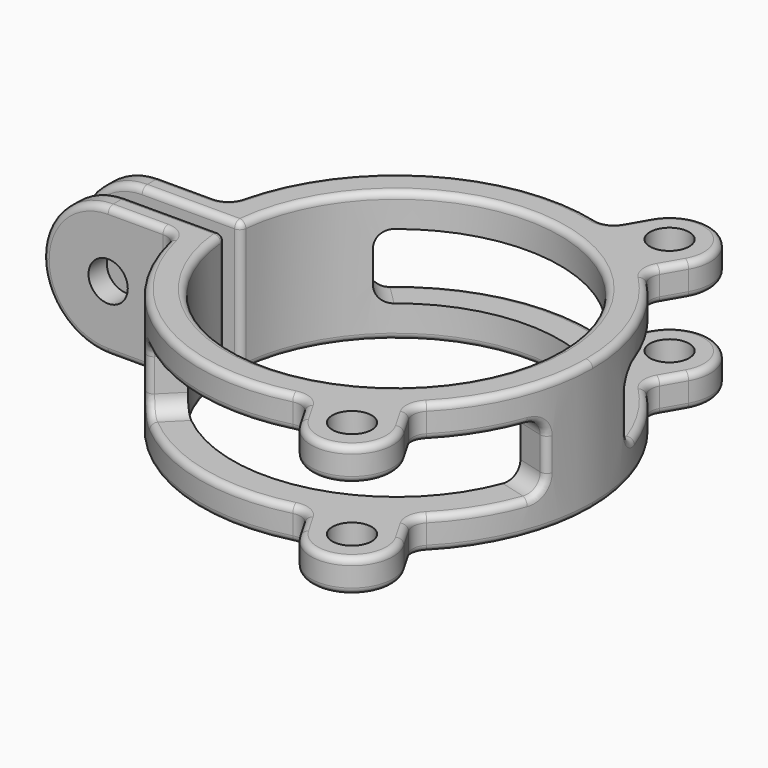
from build123d import *

# Parameters (mm, degrees)
F0_R     = 6
F1_DEPTH = 20
F2_R     = 19.99999
F3_R     = 6
F4_DEPTH = 73.1227782649
F6_DEPTH = 10
F7_R     = 5
F8_R     = 2


# Not quite as in the source:
# - a fillet or chamfer is up to 0.001 mm smaller than in the source, because OpenCascade refuses the exact size


with BuildPart() as f1:
    # F0 (on Top) → F1 (new body, symmetric)
    with BuildSketch(Plane.XY):
        with BuildLine():
            ThreePointArc((-49.76832421, 4.8076923077), (2.4066355664, 49.9420474675), (50, 0))
            Line((50, 0), (60, 0))
            ThreePointArc((60, 0), (55.5558940076, 22.6614792327), (42.8819119662, 41.9659579435))
            ThreePointArc((42.8819119662, 41.9659579435), (41.4947300268, 44.8372557208), (42.1252776112, 47.9631211055))
            Line((42.1252776112, 47.9631211055), (45.8253175473, 54.3717782649))
            ThreePointArc((45.8253175473, 54.3717782649), (41.25, 71.4470958122), (24.1746824527, 66.8717782649))
            Line((24.1746824527, 66.8717782649), (20.4746425166, 60.4631211055))
            ThreePointArc((20.4746425166, 60.4631211055), (18.0828374769, 58.3541181868), (14.9026296901, 58.1198040974))
            ThreePointArc((14.9026296901, 58.1198040974), (-31.0261270515, 51.355422695), (-58.3805106493, 13.8461538462))
            ThreePointArc((-58.3805106493, 13.8461538462), (-60.1446848386, 11.0776772972), (-63.2455532034, 10))
            Line((-63.2455532034, 10), (-100, 10))
            Line((-100, 10), (-100, 3))
            Line((-100, 3), (-51.7590571784, 3))
            ThreePointArc((-51.7590571784, 3), (-50.4145526944, 3.5193556496), (-49.76832421, 4.8076923077))
        make_face()
        with Locations((35, 60.6217782649)):
            Circle(F0_R, mode=Mode.SUBTRACT)
    extrude(amount=F1_DEPTH, both=True)

    # F2 (radius 20 in the source; OpenCascade refuses exactly that, so slightly less here)
    f2_edges = [f1.edges().sort_by_distance(p)[0] for p in [
        (-100, 6.5, 20),
        (-100, 6.5, -20),
    ]]
    fillet(f2_edges, radius=F2_R)

    # F3 (on Front) → F4 (cut, through all)
    with BuildSketch(Plane.XZ):
        with Locations((-80, 0)):
            Circle(F3_R)
    extrude(amount=-F4_DEPTH, mode=Mode.SUBTRACT)

    # F5 (on Top) → F6 (cut, symmetric)
    with BuildSketch(Plane.XY):
        with BuildLine():
            ThreePointArc((20.4746425166, 60.4631211055), (18.0828374769, 58.3541181868), (14.9026296901, 58.1198040974))
            ThreePointArc((14.9026296901, 58.1198040974), (-15.8417251808, 57.870888565), (-42.4264068712, 42.4264068712))
            Line((-42.4264068712, 42.4264068712), (-35.3553390593, 35.3553390593))
            ThreePointArc((-35.3553390593, 35.3553390593), (12.9409522551, 48.2962913145), (48.2962913145, 12.9409522551))
            Line((48.2962913145, 12.9409522551), (57.9555495773, 15.5291427062))
            ThreePointArc((57.9555495773, 15.5291427062), (52.1226890386, 29.7191064366), (42.8819119662, 41.9659579435))
            ThreePointArc((42.8819119662, 41.9659579435), (41.4947300268, 44.8372557208), (42.1252776112, 47.9631211055))
            Line((42.1252776112, 47.9631211055), (45.8253175473, 54.3717782649))
            ThreePointArc((45.8253175473, 54.3717782649), (41.25, 71.4470958122), (24.1746824527, 66.8717782649))
            Line((24.1746824527, 66.8717782649), (20.4746425166, 60.4631211055))
        make_face()
    extrude(amount=F6_DEPTH, both=True, mode=Mode.SUBTRACT)

    # F7
    f7_edges = [f1.edges().sort_by_distance(p)[0] for p in [
        (-38.890873, 38.890873, -10),
        (-38.890873, 38.890873, 10),
        (53.12592, 14.235047, 10),
        (53.12592, 14.235047, -10),
    ]]
    fillet(f7_edges, radius=F7_R)

    # F8
    f8_edges = [f1.edges().sort_by_distance(p)[0] for p in [
        (-13.414557, 58.481191, 10),
        (-31.026127, 51.355423, 20),
        (2.406636, 49.942047, 20),
    ]]
    fillet(f8_edges, radius=F8_R)

    # F9: F1 across plane


with BuildPart() as f1_1:
    add(f1.part)
    add(f1.part.mirror(Plane.XZ))


solid = f1_1.part
